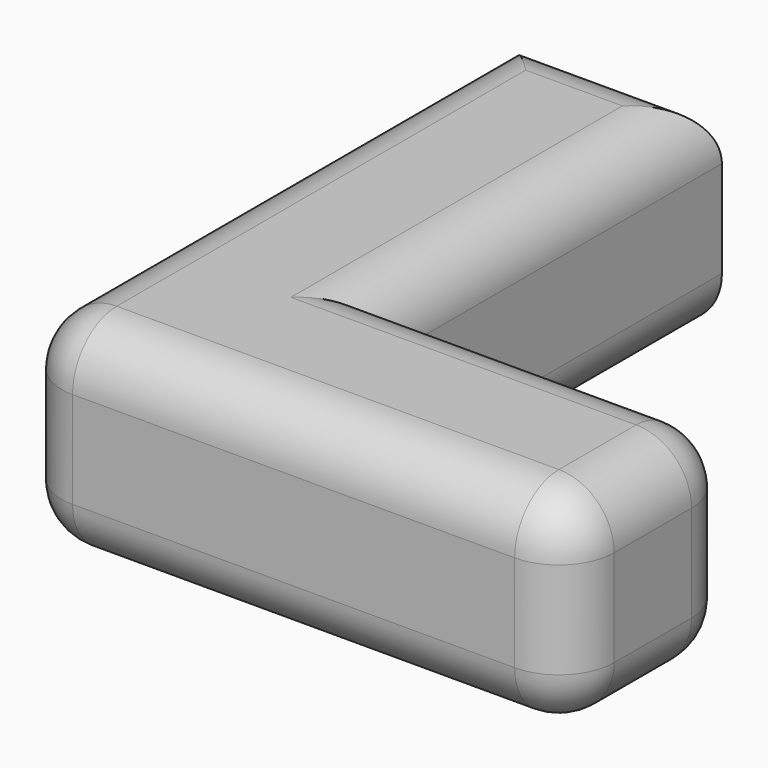
from build123d import *

# Parameters (mm, degrees)
F0_W     = 19.05
F0_H     = 57.15
F1_DEPTH = 9.525
F2_W     = 19.05
F2_H     = 19.05
F3_DEPTH = 31.75
F4_R     = 5.08


with BuildPart() as f1:
    # F0 (on Top) → F1 (new body, symmetric)
    with BuildSketch(Plane.XY):
        Rectangle(F0_W, F0_H)
    extrude(amount=F1_DEPTH, both=True)

    # F2 (on face) → F3 (join)
    with BuildSketch(Plane.YZ.offset(9.525)):
        with Locations((-19.05, 0)):
            Rectangle(F2_W, F2_H)
    extrude(amount=F3_DEPTH)

    # F4
    f4_edges = [f1.edges().sort_by_distance(p)[0] for p in [
        (9.525, 9.525, 9.525),
        (15.875, -28.575, 9.525),
        (41.275, -19.05, 9.525),
        (25.4, -9.525, 9.525),
        (0, 28.575, 9.525),
        (-9.525, 0, 9.525),
        (15.875, -28.575, -9.525),
        (41.275, -28.575, 0),
        (41.275, -9.525, 0),
        (41.275, -19.05, -9.525),
        (-9.525, 0, -9.525),
        (-9.525, -28.575, 0),
        (9.525, 9.525, -9.525),
        (25.4, -9.525, -9.525),
    ]]
    fillet(f4_edges, radius=F4_R)


solid = f1.part
